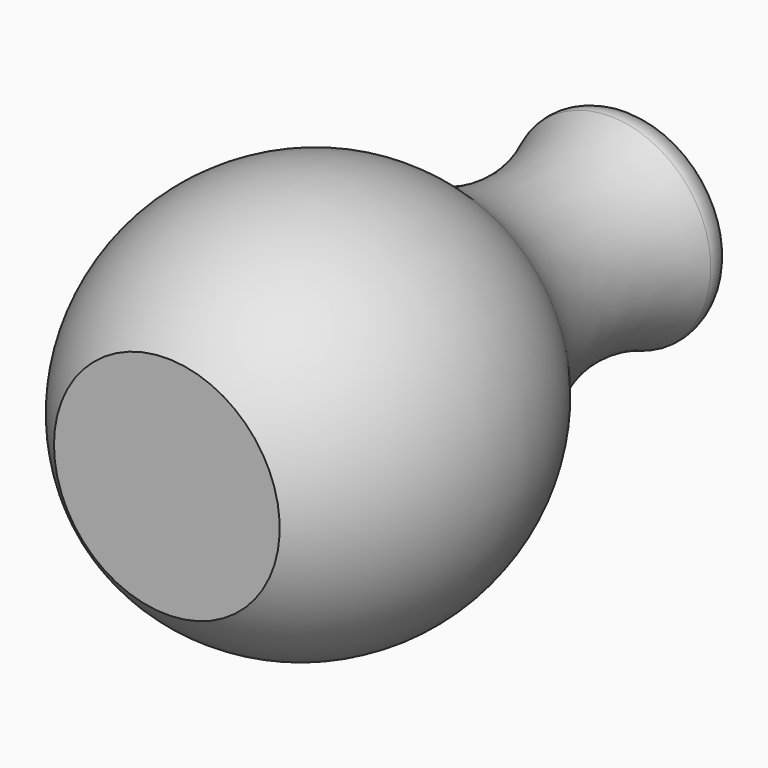
from build123d import *

# Parameters (mm, degrees)
F2_T = -2.54


# Not quite as in the source:
# - a fillet or chamfer that OpenCascade refuses, or shapes differently, is made with other operations: its cross-section is extruded or revolved along the edge and cut away or added


with BuildPart() as f1:
    # F0 (on Top) → F1 (revolve)
    with BuildSketch(Plane.XY):
        with BuildLine():
            ThreePointArc((-3.7520697053, -8.219200193), (-11.8060452517, -31.5469527597), (0, -53.2187744975))
            Line((0, -53.2187744975), (15.4842203483, -53.2187744975))
            Line((15.4842203483, -53.2187744975), (15.4842203483, 26.0937592374))
            Line((15.4842203483, 26.0937592374), (0, 26.063863188))
            ThreePointArc((0, 26.063863188), (3.7955176624, 8.3016150774), (-3.7520697053, -8.219200193))
        make_face()
    revolve(axis=Axis((15.4842203483, -13.5625076301, 0), (0, 1, 0)))

    # F2
    f2_openings = [f1.faces().sort_by_distance(p)[0] for p in [
        (23.226331, 26.078811, 0),
    ]]
    offset(amount=F2_T, openings=f2_openings, kind=Kind.INTERSECTION)

    # F3: fillet of radius 2.54 on 1 edges, made by hand

    # F3_s1 → F3_t2 (revolve, cut)
    with BuildSketch(Plane.XY):
        with BuildLine():
            add(Edge.make_bspline(
                [(1.653655928, 22.77923351), (0.6974899048, 25.0234574371), (2.9012737173, 26.0694648018)],
                knots=[0, 0, 0, 1, 1, 1], degree=2, weights=[1, 0.4285714286, 1]))
            Line((2.9012737173, 26.0694648018), (0, 26.063863188))
            ThreePointArc((0, 26.063863188), (0.8791048101, 24.4478672722), (1.653655928, 22.77923351))
        make_face()
    revolve(axis=Axis((15.4842203483, 26.063863188, 0), (0, 1, 0)), mode=Mode.SUBTRACT)


solid = f1.part
